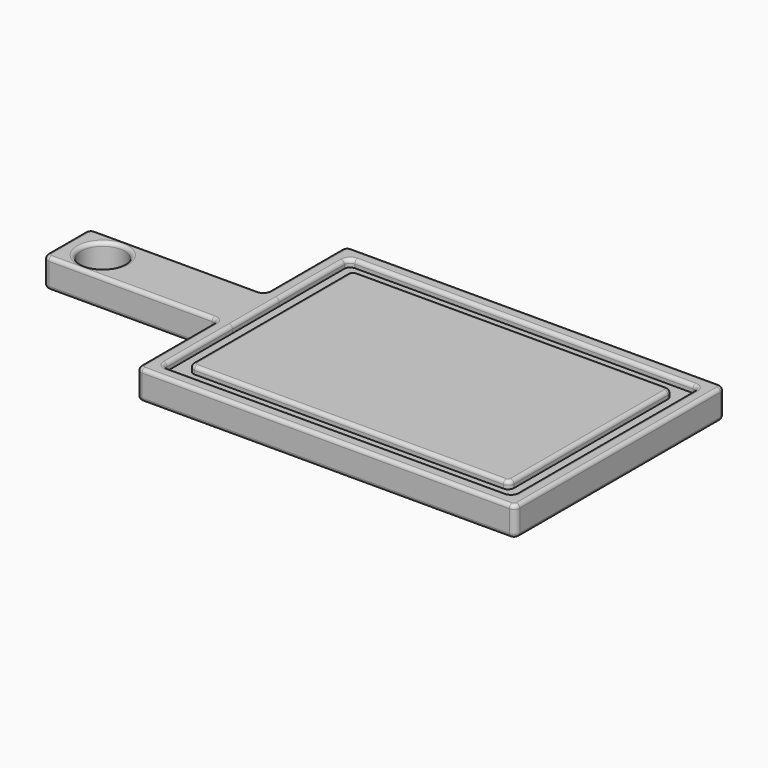
from build123d import *

# Parameters (mm, degrees)
F0_W     = 152.4
F0_H     = 50.8
F1_DEPTH = 25.4
F2_R     = 19.05
F3_DEPTH = 25.4
F5_DEPTH = 6.35
F6_R     = 5.08
F7_R     = 5.08
F8_R     = 5.08
F9_R     = 3.17499


# Not quite as in the source:
# - a fillet or chamfer is up to 0.001 mm smaller than in the source, because OpenCascade refuses the exact size
# - ends of sketch curves that miss each other by under 0.0002 mm in the source are joined


with BuildPart() as f1:
    # F0 (on Top) → F1 (new body)
    with BuildSketch(Plane.XY):
        Polygon((0, 88.9), (0, 0), (330.2, 0), (330.2, 228.6), (0, 228.6), (0, 139.7), align=None)
        with Locations((-76.2, 114.3)):
            Rectangle(F0_W, F0_H)
    extrude(amount=F1_DEPTH)

    # F2 (on face) → F3 (cut)
    with BuildSketch(Plane.XY.offset(25.4)):
        with Locations((-120.65, 114.3)):
            Circle(F2_R)
    extrude(amount=-F3_DEPTH, mode=Mode.SUBTRACT)

    # F4 (on face) → F5 (cut)
    with BuildSketch(Plane.XY.offset(25.4)):
        Polygon((12.6999960899, 215.9000039101), (12.6999960899, 139.7), (12.7, 88.9), (12.7, 12.7), (317.5, 12.7), (317.5, 215.9), align=None)
        Polygon((304.8, 25.4), (25.4, 25.4), (25.4, 88.9), (25.3999960899, 139.7), (25.3999960899, 203.2), (304.8, 203.2), align=None, mode=Mode.SUBTRACT)
    extrude(amount=-F5_DEPTH, mode=Mode.SUBTRACT)

    # F6
    f6_edges = [f1.edges().sort_by_distance(p)[0] for p in [
        (12.7, 12.7, 22.225),
        (12.699996, 215.900004, 22.225),
        (317.5, 12.7, 22.225),
        (317.5, 215.9, 22.225),
    ]]
    fillet(f6_edges, radius=F6_R)

    # F7
    f7_edges = [f1.edges().sort_by_distance(p)[0] for p in [
        (0, 228.6, 12.7),
        (0, 0, 12.7),
        (-152.4, 88.9, 12.7),
        (-152.4, 139.7, 12.7),
        (0, 139.7, 12.7),
        (0, 88.9, 12.7),
        (330.2, 0, 12.7),
        (330.2, 228.6, 12.7),
    ]]
    fillet(f7_edges, radius=F7_R)

    # F8
    f8_edges = [f1.edges().sort_by_distance(p)[0] for p in [
        (25.399996, 203.2, 22.225),
        (25.4, 25.4, 22.225),
        (304.8, 25.4, 22.225),
        (304.8, 203.2, 22.225),
    ]]
    fillet(f8_edges, radius=F8_R)

    # F9 (radius 3.175 in the source; OpenCascade refuses exactly that, so slightly less here)
    f9_edges = [f1.edges().sort_by_distance(p)[0] for p in [
        (0, 44.45, 25.4),
        (-1.487898, 87.412102, 25.4),
        (1.487898, 1.487898, 25.4),
        (-76.2, 88.9, 25.4),
        (165.1, 0, 25.4),
        (-150.912102, 90.387898, 25.4),
        (328.712102, 1.487898, 25.4),
        (-152.4, 114.3, 25.4),
        (330.2, 114.3, 25.4),
        (-150.912102, 138.212102, 25.4),
        (328.712102, 227.112102, 25.4),
        (-76.2, 139.7, 25.4),
        (165.1, 228.6, 25.4),
        (-1.487898, 141.187898, 25.4),
        (1.487898, 227.112102, 25.4),
        (0, 184.15, 25.4),
        (12.699996, 175.260002, 25.4),
        (14.187894, 214.412106, 25.4),
        (12.699998, 114.3, 25.4),
        (165.099998, 215.900002, 25.4),
        (12.7, 53.34, 25.4),
        (316.012102, 214.412102, 25.4),
        (14.187898, 14.187898, 25.4),
        (317.5, 114.3, 25.4),
        (165.1, 12.7, 25.4),
        (316.012102, 14.187898, 25.4),
        (-139.7, 114.3, 25.4),
        (165.1, 25.4, 25.4),
        (303.312102, 26.887898, 25.4),
        (26.887898, 26.887898, 25.4),
        (304.8, 114.3, 25.4),
        (25.4, 59.69, 25.4),
        (303.312102, 201.712102, 25.4),
        (25.399998, 114.3, 25.4),
        (165.099998, 203.2, 25.4),
        (25.399996, 168.91, 25.4),
        (26.887894, 201.712102, 25.4),
        (0, 44.45, 0),
        (-1.487898, 87.412102, 0),
        (1.487898, 1.487898, 0),
        (-76.2, 88.9, 0),
        (165.1, 0, 0),
        (-150.912102, 90.387898, 0),
        (328.712102, 1.487898, 0),
        (-152.4, 114.3, 0),
        (330.2, 114.3, 0),
        (-150.912102, 138.212102, 0),
        (328.712102, 227.112102, 0),
        (-76.2, 139.7, 0),
        (165.1, 228.6, 0),
        (-1.487898, 141.187898, 0),
        (1.487898, 227.112102, 0),
        (0, 184.15, 0),
        (-139.7, 114.3, 0),
    ]]
    fillet(f9_edges, radius=F9_R)


solid = f1.part
